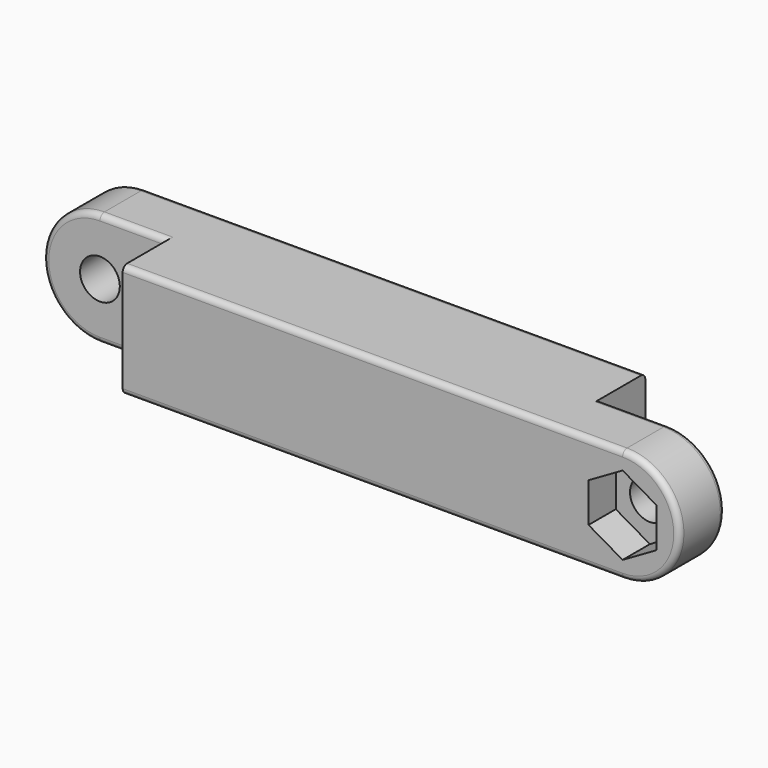
from build123d import *

# Parameters (mm, degrees)
F0_W     = 50
F0_H     = 10
F1_DEPTH = 10
F2_W     = 13.4624946701
F2_H     = 5
F2_W_2   = 13.2752915323
F3_DEPTH = 25
F4_R     = 1.75
F5_DEPTH = 25
F7_DEPTH = 3
F8_R     = 0.5


# Not quite as in the source:
# - a feature names something its author has since deleted; it is built from what else it names


with BuildPart() as f1:
    # F0 (on Front) → F1 (new body)
    with BuildSketch(Plane.XZ):
        with Locations((25, 5)):
            Rectangle(F0_W, F0_H)
        with BuildLine():
            ThreePointArc((0, 10), (-5, 5), (0, 0))
            Line((0, 0), (0, 10))
        make_face()
        with BuildLine():
            Line((50, 10), (50, 0))
            ThreePointArc((50, 0), (55, 5), (50, 10))
        make_face()
    extrude(amount=F1_DEPTH)

    # F2 (on face) → F3 (cut)
    with BuildSketch(Plane.XY.offset(10)):
        with Locations((-0.7312473351, -7.5)):
            Rectangle(F2_W, F2_H)
        with Locations((50.6376457661, -2.5)):
            Rectangle(F2_W_2, F2_H)
    extrude(amount=-F3_DEPTH, mode=Mode.SUBTRACT)

    # F4 (on face) → F5 (cut)
    with BuildSketch(Plane.XZ.offset(10)):
        with Locations((50, 5)):
            Circle(F4_R)
        with Locations((0, 5)):
            Circle(F4_R)
    extrude(amount=-F5_DEPTH, mode=Mode.SUBTRACT)

    # F6 (on face) → F7 (cut)
    with BuildSketch(Plane.XZ.offset(10)):
        Polygon((53, 3.2679491924), (53, 6.7320508076), (50, 8.4641016151), (47, 6.7320508076), (47, 3.2679491924), (50, 1.5358983849), align=None)
    extrude(amount=-F7_DEPTH, mode=Mode.SUBTRACT)

    # F8
    f8_edges = [f1.edges().sort_by_distance(p)[0] for p in [
        (28, -10, 10),
        (22, 0, 10),
        (-5, -5, 5),
        (55, -5, 5),
        (22, 0, 0),
        (47, -5, 0),
        (28, -10, 0),
        (3, -5, 0),
        (-5, 0, 5),
        (47, -5, 10),
        (55, -10, 5),
        (3, -5, 10),
    ]]
    fillet(f8_edges, radius=F8_R)


solid = f1.part
